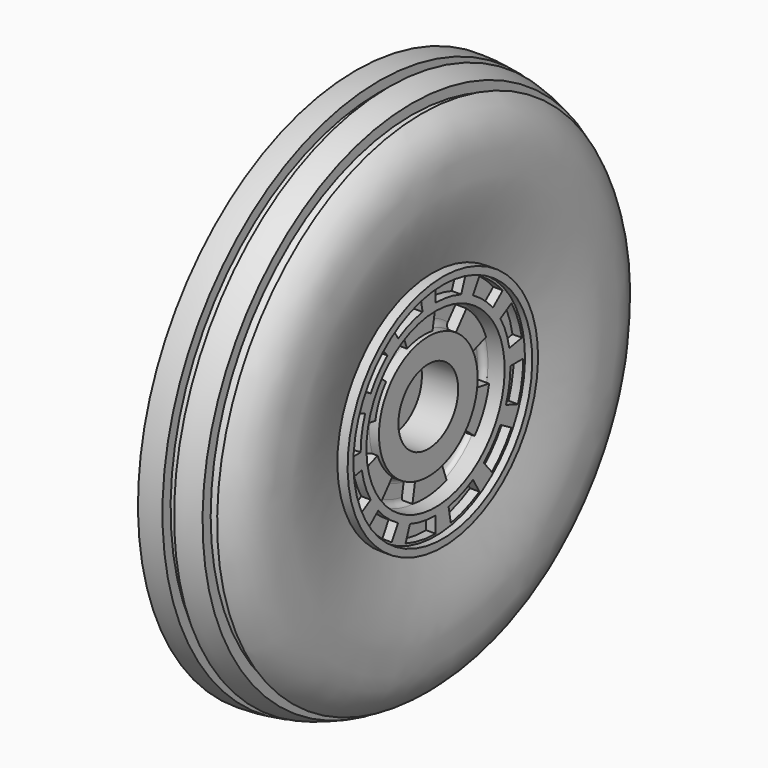
from build123d import *

# Parameters (mm, degrees)
F2_W            = 0.2
F2_H            = 0.22
F3_ANGLE        = 20
F3_COPIES_COUNT = 12
F5_DEPTH        = 0.15


# Not quite as in the source:
# - a pattern or mirror of a feature is missing from the dataset's text; its kind, count and spacing are read off the source's solid


with BuildPart() as f1:
    # F0 (on Front) → F1 (revolve)
    with BuildSketch(Plane.XZ):
        with BuildLine():
            Line((1, 0.85), (0.87, 0.85))
            ThreePointArc((0.87, 0.85), (0.8134314575, 0.8734314575), (0.79, 0.93))
            Line((0.79, 0.93), (0.79, 1.11))
            ThreePointArc((0.79, 1.11), (0.8134314575, 1.1665685425), (0.87, 1.19))
            Line((0.87, 1.19), (1.1, 1.19))
            Line((1.1, 1.19), (1.1, 1.54))
            Line((1.1, 1.54), (1.2, 1.54))
            Line((1.2, 1.54), (1.2, 1.64))
            Line((1.2, 1.64), (1.12, 1.64))
            Line((1.12, 1.64), (1.0590550792, 1.64))
            add(Edge.make_bspline(
                [(1.0590550792, 1.64), (1.25, 2.3421209771), (1.2635455001, 2.685534462), (1.2259744013, 3.2558219262), (0.9930693577, 3.4693235058), (0.91, 3.5233867214)],
                knots=[0, 0, 0, 0, 0.3714125336, 0.6273384476, 0.7316891336, 0.7316891336, 0.7316891336, 0.7316891336], degree=3))
            Line((0.91, 3.5233867214), (0.91, 3.3833867214))
            Line((0.91, 3.3833867214), (0.77, 3.4602341654))
            Line((0.77, 3.4602341654), (0.77, 3.6002341654))
            add(Edge.make_bspline(
                [(0.77, 3.6002341654), (0.6784642229, 3.6425426702), (0.5744947558, 3.6771881754), (0.46, 3.7024604996)],
                knots=[0.7852748547, 0.7852748547, 0.7852748547, 0.7852748547, 0.8822719118, 0.8822719118, 0.8822719118, 0.8822719118], degree=3))
            Line((0.46, 3.7024604996), (0.46, 3.5624604996))
            Line((0.46, 3.5624604996), (0.32, 3.5878456739))
            Line((0.32, 3.5878456739), (0.32, 3.7278456739))
            add(Edge.make_bspline(
                [(0.32, 3.7278456739), (0.2195553432, 3.7423008552), (0.1125378698, 3.75), (0, 3.75)],
                knots=[0.9204576606, 0.9204576606, 0.9204576606, 0.9204576606, 1, 1, 1, 1], degree=3))
            Line((0, 3.75), (0, 2.75))
            Line((0, 2.75), (0, 2.5))
            Line((0, 2.5), (-0.35, 2.5))
            Line((-0.35, 2.5), (-0.35, 2.2))
            Line((-0.35, 2.2), (0.02, 2.2))
            Line((0.02, 2.2), (0.02, 2.15))
            Line((0.02, 2.15), (0.02, 0))
            Line((0.02, 0), (0.5, 0))
            Line((0.5, 0), (0.5, 0.515))
            Line((0.5, 0.515), (1, 0.515))
            Line((1, 0.515), (1, 0.85))
        make_face()
    revolve(axis=Axis((1.052, 0, 0), (1, 0, 0)))

    # F2 (on Front) → F3 (revolve, cut)
    with BuildSketch(Plane.XZ):
        with Locations((1.07, 1.4)):
            Rectangle(F2_W, F2_H)
    f3 = revolve(axis=Axis((1.36, 0, 0), (-1, 0, 0)), revolution_arc=F3_ANGLE, mode=Mode.SUBTRACT)

    # F3_copies: F3 ×12 about axis
    f3_copies_axis = Axis((0, 0, 0), (1, 0, 0))
    for i in range(1, F3_COPIES_COUNT):
        add(f3.rotate(f3_copies_axis, i * 360 / F3_COPIES_COUNT), mode=Mode.SUBTRACT)

    # F4 (on face) → F5 (join)
    with BuildSketch(Plane.YZ.offset(0.79)):
        with BuildLine():
            Line((-0.3895609432, 1.0703098951), (-0.2696546218, 0.7408699845))
            ThreePointArc((-0.2696546218, 0.7408699845), (-0.0687151015, 0.7854172037), (0.1369072395, 0.7764395384))
            Line((0.1369072395, 0.7764395384), (0.1977852744, 1.1216960307))
            ThreePointArc((0.1977852744, 1.1216960307), (-0.099270391, 1.1346657611), (-0.3895609432, 1.0703098951))
        make_face()
        with BuildLine():
            Line((-1.1216960307, 0.1977852744), (-0.7764395384, 0.1369072395))
            ThreePointArc((-0.7764395384, 0.1369072395), (-0.7145488017, 0.3331995784), (-0.603962745, 0.5067849166))
            Line((-0.603962745, 0.5067849166), (-0.8725246207, 0.7321350874))
            ThreePointArc((-0.8725246207, 0.7321350874), (-1.0322845694, 0.4813622001), (-1.1216960307, 0.1977852744))
        make_face()
        with BuildLine():
            Line((-0.7321350874, -0.8725246207), (-0.5067849166, -0.603962745))
            ThreePointArc((-0.5067849166, -0.603962745), (-0.6458337002, -0.4522176253), (-0.7408699845, -0.2696546218))
            Line((-0.7408699845, -0.2696546218), (-1.0703098951, -0.3895609432))
            ThreePointArc((-1.0703098951, -0.3895609432), (-0.9330141784, -0.653303561), (-0.7321350874, -0.8725246207))
        make_face()
        with BuildLine():
            Line((0.3895609432, -1.0703098951), (0.2696546218, -0.7408699845))
            ThreePointArc((0.2696546218, -0.7408699845), (0.0687151015, -0.7854172037), (-0.1369072395, -0.7764395384))
            Line((-0.1369072395, -0.7764395384), (-0.1977852744, -1.1216960307))
            ThreePointArc((-0.1977852744, -1.1216960307), (0.099270391, -1.1346657611), (0.3895609432, -1.0703098951))
        make_face()
        with BuildLine():
            Line((1.1216960307, -0.1977852744), (0.7764395384, -0.1369072395))
            ThreePointArc((0.7764395384, -0.1369072395), (0.7145488017, -0.3331995784), (0.603962745, -0.5067849166))
            Line((0.603962745, -0.5067849166), (0.8725246207, -0.7321350874))
            ThreePointArc((0.8725246207, -0.7321350874), (1.0322845694, -0.4813622001), (1.1216960307, -0.1977852744))
        make_face()
        with BuildLine():
            Line((0.7321350874, 0.8725246207), (0.5067849166, 0.603962745))
            ThreePointArc((0.5067849166, 0.603962745), (0.6458337002, 0.4522176253), (0.7408699845, 0.2696546218))
            Line((0.7408699845, 0.2696546218), (1.0703098951, 0.3895609432))
            ThreePointArc((1.0703098951, 0.3895609432), (0.9330141784, 0.653303561), (0.7321350874, 0.8725246207))
        make_face()
    extrude(amount=F5_DEPTH)


solid = f1.part
